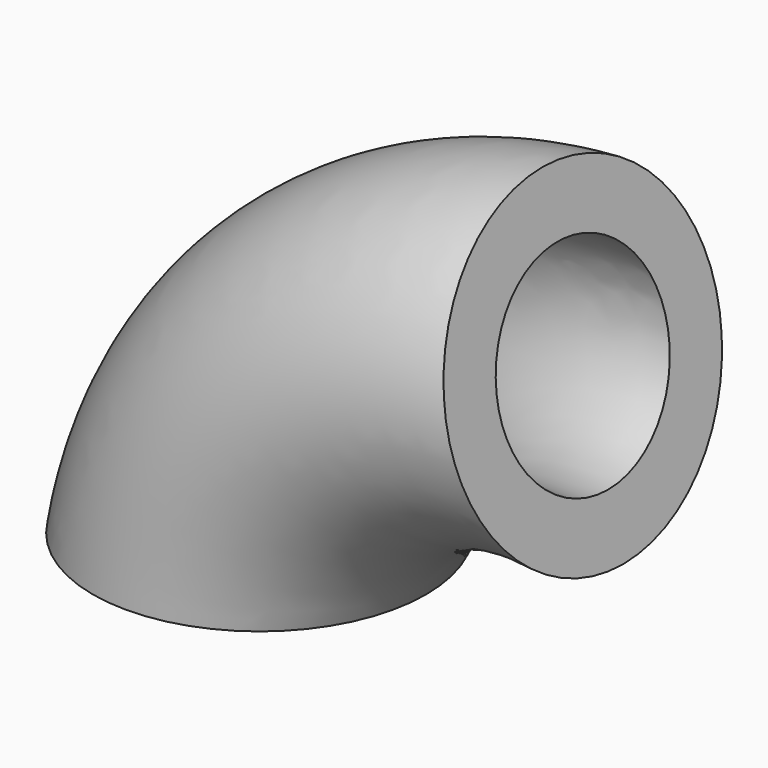
from build123d import *

# Parameters (mm, degrees)
F1_R   = 12.7
F1_R_2 = 7.9375


with BuildPart() as f2:
    # F2: sweep along a path in F0
    with BuildLine(Plane.XZ) as f2_path:
        ThreePointArc((24.6416195037, 19.2395951241), (9.0101493849, 13.8600132497), (0, 0))
    # F1 (on Top) → F2 (sweep)
    with BuildSketch(Plane.XY):
        Circle(F1_R)
        Circle(F1_R_2, mode=Mode.SUBTRACT)
    sweep(path=f2_path.line)


solid = f2.part
